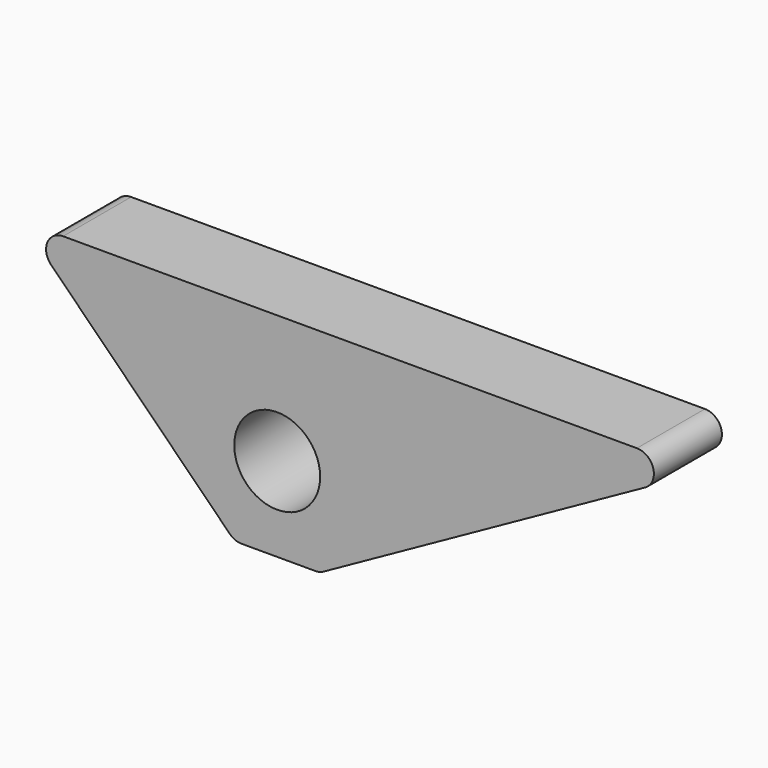
from build123d import *

# Parameters (mm, degrees)
F2_DEPTH = 25.4
F3_DEPTH = 25.4
F4_R     = 5.08
F5_R     = 12.827
F5_R_2   = 12.7
F6_DEPTH = 25.4


with BuildPart() as f2:
    # F0 (on Front) → F2 (new body)
    with BuildSketch(Plane.XZ):
        Polygon((-12.7, -16.6841130704), (0, -16.6841130704), (0, 46.8158869296), (-76.2, 46.8158869296), align=None)
        Polygon((0, 46.8158869296), (0, -16.6841130704), (12.7, -16.6841130704), (127, 46.8158869296), align=None)
    extrude(amount=F2_DEPTH)

    # F1 (on face) → F3 (cut)
    with BuildSketch(Plane.XZ):
        with BuildLine():
            ThreePointArc((0, 21.231531626), (-12.7, 8.531531626), (0, -4.168468374))
            Line((0, -4.168468374), (0, 8.531531626))
            Line((0, 8.531531626), (0, 21.231531626))
        make_face()
        with BuildLine():
            Line((0, 8.531531626), (0, -4.168468374))
            ThreePointArc((0, -4.168468374), (8.9802561211, -0.4487244951), (12.7, 8.531531626))
            ThreePointArc((12.7, 8.531531626), (8.9802561211, 17.5117877471), (0, 21.231531626))
            Line((0, 21.231531626), (0, 8.531531626))
        make_face()
    extrude(amount=F3_DEPTH, mode=Mode.SUBTRACT)

    # F4
    f4_edges = [f2.edges().sort_by_distance(p)[0] for p in [
        (-12.7, -12.7, -16.684113),
        (12.7, -12.7, -16.684113),
        (127, -12.7, 46.815887),
        (-76.2, -12.7, 46.815887),
    ]]
    fillet(f4_edges, radius=F4_R)

    # F5 (on face) → F6 (cut)
    with BuildSketch(Plane.XZ.offset(25.4)):
        with Locations((0, 8.531531626)):
            Circle(F5_R)
        with Locations((0, 8.531531626)):
            Circle(F5_R_2, mode=Mode.SUBTRACT)
    extrude(amount=-F6_DEPTH, mode=Mode.SUBTRACT)


solid = f2.part
